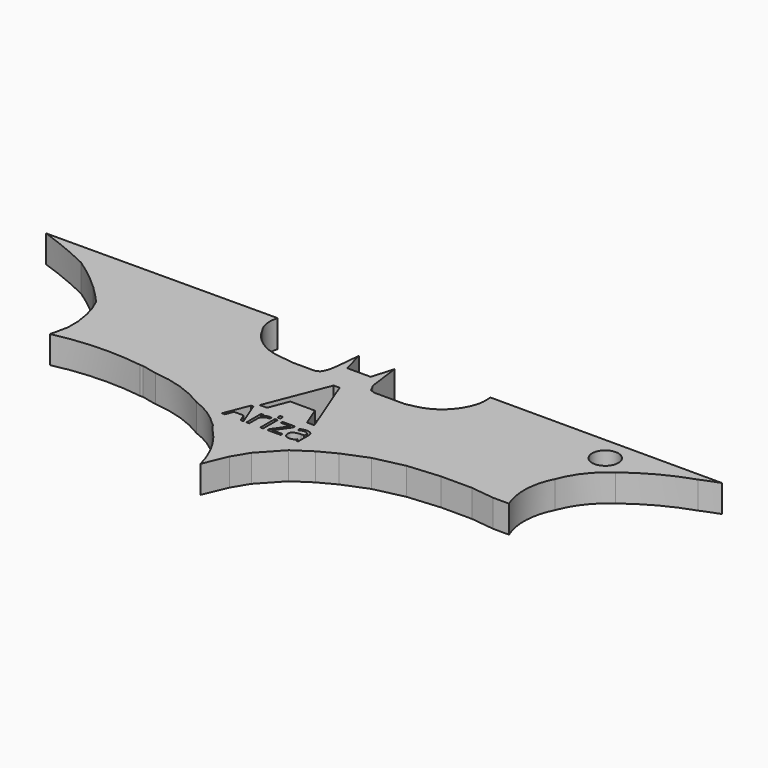
from build123d import *

# Parameters (mm, degrees)
F1_DEPTH      = 4
F3_DEPTH      = 25
F5_DEPTH      = 25
F7_DEPTH      = 25
F9_DEPTH      = 25
F11_DEPTH     = 25
F13_DEPTH     = 25
F14_TEXT_SIZE = 12.6210106019
F15_DEPTH     = 25
F17_DEPTH     = 25
F18_R         = 1.91377607
F19_DEPTH     = 25
F20_TEXT_SIZE = 4.9846997071
F21_DEPTH     = 25
F23_DEPTH     = 25
F25_DEPTH     = 25


# Not quite as in the source:
# - Text() gives the source's letters only with a copy of the font that has no kerning and outlines rounded to 1/6400 em; it was checked with that copy


with BuildPart() as f1:
    # F0 (on Top) → F1 (new body)
    with BuildSketch(Plane.XY):
        Polygon((13.7181449682, 28.8296956569), (13.7181449682, 31.2483999878), (-20.0392529368, 31.1019383371), (-15.5726019293, 29.3966997415), (-12.4151417986, 27.9607102275), (-10.6438836083, 26.5457220376), (-9.2191752046, 25.5693010986), (-7.44791748, 24.0066461265), (-6.4045181498, 22.9374337941), (-5.0068260004, 21.443657577), (-4.050786607, 18.9938060939), (-3.5693414975, 16.4260994643), (-3.5693414975, 14.446824789), (-4.157774616, 11.9246225804), (-0.9481405723, 12.4065233395), (2.3816456087, 12.4065233395), (5.301555153, 12.4065233395), (9.1226715595, 12.4065233395), (11.2855676562, 11.9246225804), (14.2415259033, 11.2890275195), (17.4137726426, 10.2436281741), (20.4586461186, 8.7500112131), (22.4141739309, 7.4366261251), (24.3864022195, 6.0528814793), (26.0066930205, 3.9328928106), (27.5012981147, 1.9948538393), (29.3448008597, -2.4011868518), (30.8101475239, 1.0967379203), (32.1809537709, 3.3656621817), (35.1002141833, 6.5197809599), (37.6546531916, 8.2134958357), (40.1031784713, 9.5021920279), (43.678548187, 10.9441205859), (48.0499491096, 11.9246225804), (52.7073331177, 12.3331649229), (57.2421513498, 12.3331649229), (60.6739073992, 11.9246225804), (63.0025938153, 11.9246225804), (62.512345612, 15.3972320259), (62.512345612, 17.766777426), (63.3294284344, 19.9729055166), (64.0648081899, 21.443657577), (65.177924931, 22.9374337941), (67.6972419024, 25.5693010986), (70.7145631313, 27.5073572993), (73.4975337982, 29.0306657553), (78.8051709533, 31.1019383371), (44.9277721345, 31.1019383371), (44.9277721345, 29.3966997415), (44.4790236652, 27.9607102275), (43.5815304518, 26.5457220376), (42.7289120853, 25.5693010986), (41.1134213209, 25.0281393528), (39.5876839757, 24.0066461265), (38.196567446, 23.7321238965), (36.6708263755, 23.7321238965), (35.1002141833, 23.7321238965), (33.7539725006, 23.7321238965), (33.1675857306, 24.0066461265), (32.6368100941, 25.0281393528), (32.0175737143, 29.7507476062), (31.0887135565, 26.5457220376), (29.8198983073, 26.5457220376), (27.6577975601, 26.5457220376), (26.7782844603, 29.7507476062), (26.6447421163, 28.2817762345), (26.4730453491, 26.5457220376), (26.3395030051, 25.5693010986), (26.2371003628, 25.0281393528), (26.0066930205, 24.4501009583), (25.7506873459, 24.0066461265), (25.1888465136, 23.7321238965), (24.3864022195, 23.7321238965), (23.6261896789, 23.7321238965), (21.9579506665, 23.7321238965), (20.4586461186, 24.0066461265), (18.9804602414, 24.4501009583), (17.6289733499, 24.9146744609), (16.1296706647, 25.5693010986), (14.9471201003, 26.8152002245), (14.2502607778, 27.7654640377), align=None)
    extrude(amount=F1_DEPTH)

    # F2 (on face) → F3 (cut)
    with BuildSketch(Plane.XY.offset(4)):
        with BuildLine():
            ThreePointArc((39.5876839757, 24.0066461265), (42.5224022258, 25.378705214), (44.4790236652, 27.9607102275))
            ThreePointArc((44.4790236652, 27.9607102275), (44.9430916505, 29.4970821961), (44.9277721345, 31.1019383371))
            Line((44.9277721345, 31.1019383371), (38.196567446, 23.7321238965))
            ThreePointArc((38.196567446, 23.7321238965), (38.8941668952, 23.8590414949), (39.5876839757, 24.0066461265))
        make_face()
    extrude(amount=-F3_DEPTH, mode=Mode.SUBTRACT)

    # F4 (on face) → F5 (cut)
    with BuildSketch(Plane.XY.offset(4)):
        with BuildLine():
            Line((20.4586461186, 24.0066461265), (13.7181449682, 31.2483999878))
            ThreePointArc((13.7181449682, 31.2483999878), (13.5730980502, 29.4441242613), (14.2502607778, 27.7654640377))
            ThreePointArc((14.2502607778, 27.7654640377), (16.8112352565, 24.9888294281), (20.4586461186, 24.0066461265))
        make_face()
    extrude(amount=-F5_DEPTH, mode=Mode.SUBTRACT)

    # F6 (on face) → F7 (cut)
    with BuildSketch(Plane.XY.offset(4)):
        Polygon((19.5419695228, 24.8886570334), (19.3606550324, 24.075507841), (21.9579506665, 23.7321238965), (21.9579506665, 24.8886570334), align=None)
    extrude(amount=-F7_DEPTH, mode=Mode.SUBTRACT)

    # F8 (on face) → F9 (cut)
    with BuildSketch(Plane.XY.offset(4)):
        with BuildLine():
            Line((-20.0392529368, 31.1019383371), (-4.157774616, 11.9246225804))
            ThreePointArc((-4.157774616, 11.9246225804), (-3.6491679308, 16.7673709248), (-5.0068260004, 21.443657577))
            ThreePointArc((-5.0068260004, 21.443657577), (-8.4946034862, 24.948156203), (-12.4151417986, 27.9607102275))
            ThreePointArc((-12.4151417986, 27.9607102275), (-16.1783838461, 29.649800146), (-20.0392529368, 31.1019383371))
        make_face()
    extrude(amount=-F9_DEPTH, mode=Mode.SUBTRACT)

    # F10 (on face) → F11 (cut)
    with BuildSketch(Plane.XY.offset(4)):
        with BuildLine():
            ThreePointArc((67.6972419024, 25.5693010986), (65.0789550784, 23.1101235179), (63.3294284344, 19.9729055166))
            ThreePointArc((63.3294284344, 19.9729055166), (62.2694629017, 15.9851721867), (63.0025938153, 11.9246225804))
            Line((63.0025938153, 11.9246225804), (78.8051709533, 31.1019383371))
            ThreePointArc((78.8051709533, 31.1019383371), (77.4718636032, 30.6005152273), (76.1513523757, 30.0663020462))
            ThreePointArc((76.1513523757, 30.0663020462), (71.7372828091, 28.1693780618), (67.6972419024, 25.5693010986))
        make_face()
    extrude(amount=-F11_DEPTH, mode=Mode.SUBTRACT)

    # F12 (on face) → F13 (cut)
    with BuildSketch(Plane.XY.offset(4)):
        with BuildLine():
            ThreePointArc((19.475884682, 9.2320900784), (15.5446276032, 11.0769221611), (11.2855676562, 11.9246225804))
            ThreePointArc((11.2855676562, 11.9246225804), (3.5638965201, 12.7744117011), (-4.157774616, 11.9246225804))
            Line((-4.157774616, 11.9246225804), (29.3448008597, -2.4011868518))
            ThreePointArc((29.3448008597, -2.4011868518), (27.7728833382, 1.5776015221), (25.19654762, 4.9928871449))
            ThreePointArc((25.19654762, 4.9928871449), (22.6450351586, 7.5292295601), (19.475884682, 9.2320900784))
        make_face()
    extrude(amount=-F13_DEPTH, mode=Mode.SUBTRACT)

    # F14 (on face) → F15 (cut)
    with BuildSketch(Plane.XY.offset(4)):
        with Locations((25.5532991141, 13.175486587)):
            Text('A', F14_TEXT_SIZE, font='Open Sans', text_align=(TextAlign.LEFT, TextAlign.BOTTOM))
    extrude(amount=-F15_DEPTH, mode=Mode.SUBTRACT)

    # F16 (on face) → F17 (cut)
    with BuildSketch(Plane.XY.offset(4)):
        Polygon((29.5112095773, 21.6882135719), (27.7225353113, 17.0550514013), (28.0205402523, 16.6118796915), (31.3333275632, 16.6118796915), (31.3333275632, 17.3773579299), align=None)
    extrude(amount=-F17_DEPTH, mode=Mode.SUBTRACT)

    # F18 (on face) → F19 (cut)
    with BuildSketch(Plane(origin=(0, 0, 0), x_dir=(1, 0, 0), z_dir=(0, 0, -1))):
        with Locations((64.5570829511, -27.5814495981)):
            Circle(F18_R)
    extrude(amount=-F19_DEPTH, mode=Mode.SUBTRACT)

    # F20 (on face) → F21 (cut)
    with BuildSketch(Plane.XY.offset(4)):
        with Locations((23.4450697899, 8.8981278241)):
            Text('Ariza', F20_TEXT_SIZE, font='Open Sans', text_align=(TextAlign.LEFT, TextAlign.BOTTOM))
    extrude(amount=-F21_DEPTH, mode=Mode.SUBTRACT)

    # F22 (on face) → F23 (cut)
    with BuildSketch(Plane.XY.offset(4)):
        Polygon((25.8588977158, 10.2366143838), (25.091715157, 12.2430901974), (24.8881216354, 12.1633479223), (24.2212601006, 10.2366143838), align=None)
    extrude(amount=-F23_DEPTH, mode=Mode.SUBTRACT)

    # F24 (on face) → F25 (cut)
    with BuildSketch(Plane.XY.offset(4)):
        Polygon((34.3658458747, 9.6357076088), (34.2051647604, 10.3739760816), (32.8266397119, 10.1845609024), (32.8266397119, 9.1743450612), (33.7485998563, 9.0270219371), align=None)
    extrude(amount=-F25_DEPTH, mode=Mode.SUBTRACT)


solid = f1.part
